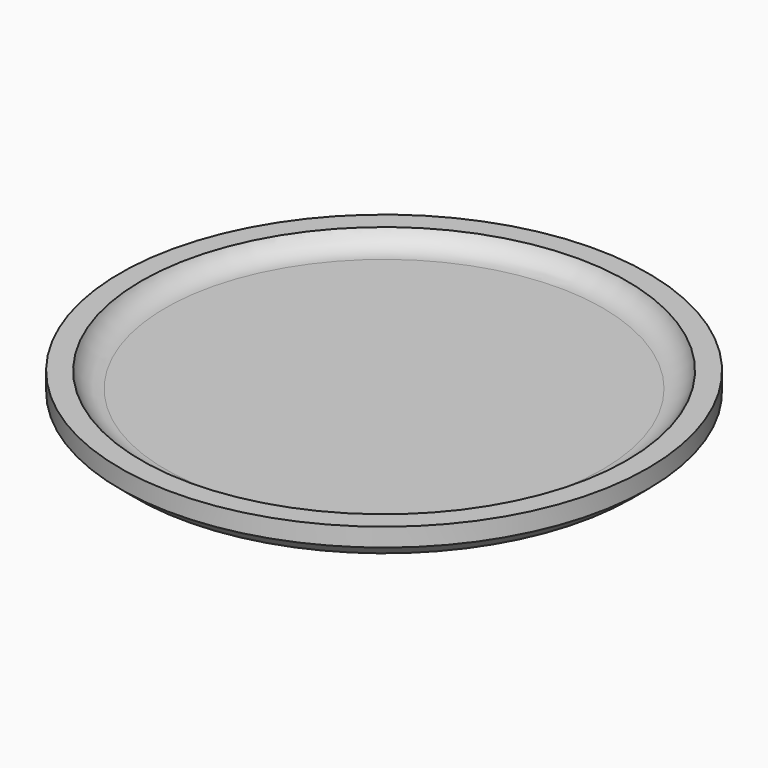
from build123d import *


# Not quite as in the source:
# - a fillet or chamfer that OpenCascade refuses, or shapes differently, is made with other operations: its cross-section is extruded or revolved along the edge and cut away or added


with BuildPart() as f1:
    # F0 (on Front) → F1 (revolve)
    with BuildSketch(Plane.XZ):
        Polygon((0, 15), (0, 0), (235, 0), (250, 12.5864944677), (250, 30), (230, 30), (230, 15), align=None)
    revolve(axis=Axis((0, 0, 7.5), (0, 0, -1)))

    # F2: fillet of radius 25 on 1 edges, made by hand

    # F2_s1 → F2_t2 (revolve)
    with BuildSketch(Plane.XZ):
        with BuildLine():
            ThreePointArc((230, 30), (220.7801854628, 19.0834993366), (207.0871215252, 15))
            Line((207.0871215252, 15), (230, 15))
            Line((230, 15), (230, 30))
        make_face()
    revolve(axis=Axis((0, 0, 15), (0, 0, -1)))


solid = f1.part
